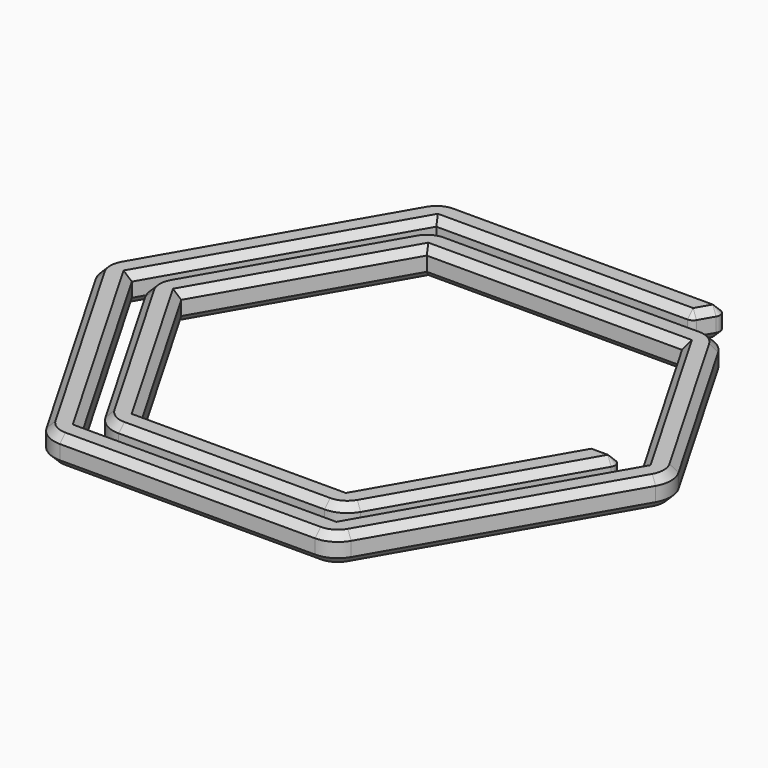
from build123d import *

# Parameters (mm, degrees)
F1_DEPTH = 2
F2_R     = 0.5
F3_R     = 2
F4_SIZE  = 0.49999


# Not quite as in the source:
# - a fillet or chamfer is up to 0.001 mm smaller than in the source, because OpenCascade refuses the exact size


with BuildPart() as f1:
    # F0 (on Top) → F1 (new body)
    with BuildSketch(Plane.XY):
        Polygon((-14.4337567297, 0), (-7.2168783649, 12.5), (7.2168783649, 12.5), (9.5262794416, 12.5), (10.68097998, 12.5), (17.8978583449, 0), (8.9489291724, -15.5), (-8.9489291724, -15.5), (-17.8978583449, 0), (-8.9489291724, 15.5), (8.9489291724, 15.5), (10.1036297108, 17.5), (-10.1036297108, 17.5), (-20.2072594216, 0), (-10.1036297108, -17.5), (10.1036297108, -17.5), (20.2072594216, 0), (11.8356805184, 14.5), (8.3715789032, 14.5), (-8.3715789032, 14.5), (-16.7431578065, 0), (-8.3715789032, -14.5), (8.3715789032, -14.5), (16.7431578065, 0), (14.4337567297, 0), (7.2168783649, -12.5), (-7.2168783649, -12.5), align=None)
    extrude(amount=F1_DEPTH)

    # F2
    f2_edges = [f1.edges().sort_by_distance(p)[0] for p in [
        (16.743158, 0, 1),
        (14.433757, 0, 1),
        (10.10363, 17.5, 1),
        (8.948929, 15.5, 1),
    ]]
    fillet(f2_edges, radius=F2_R)

    # F3
    f3_edges = [f1.edges().sort_by_distance(p)[0] for p in [
        (-10.10363, 17.5, 1),
        (-20.207259, 0, 1),
        (-10.10363, -17.5, 1),
        (10.10363, -17.5, 1),
        (20.207259, 0, 1),
        (11.835681, 14.5, 1),
        (-8.371579, 14.5, 1),
        (-16.743158, 0, 1),
        (-8.371579, -14.5, 1),
        (8.371579, -14.5, 1),
    ]]
    fillet(f3_edges, radius=F3_R)

    # F4 (size 0.5 in the source; OpenCascade refuses exactly that, so slightly less here)
    f4_edges = [f1.edges().sort_by_distance(p)[0] for p in [
        (12.629537, -7.125, 0),
        (8.216878, -14.232051, 0),
        (16.310145, -0.25, 0),
        (0, -14.5, 0),
        (15.299782, 0, 0),
        (-8.216878, -14.232051, 0),
        (14.472432, -0.066987, 0),
        (-12.557368, -7.25, 0),
        (10.753149, -6.375, 0),
        (-16.433757, 0, 0),
        (0, -12.5, 0),
        (-12.557368, 7.25, 0),
        (-10.825318, -6.25, 0),
        (-8.216878, 14.232051, 0),
        (-10.825318, 6.25, 0),
        (1.732051, 14.5, 0),
        (1.732051, 12.5, 0),
        (11.68098, 14.232051, 0),
        (14.289419, 6.25, 0),
        (16.02147, 7.25, 0),
        (13.423394, -7.75, 0),
        (19.897858, 0, 0),
        (0, -15.5, 0),
        (15.155445, -8.75, 0),
        (-13.423394, -7.75, 0),
        (9.948929, -17.232051, 0),
        (-13.423394, 7.75, 0),
        (0, -17.5, 0),
        (-0.144338, 15.5, 0),
        (-9.948929, -17.232051, 0),
        (8.910254, 15.566987, 0),
        (-15.155445, -8.75, 0),
        (9.381942, 16.25, 0),
        (-19.897858, 0, 0),
        (9.670617, 17.25, 0),
        (-15.155445, 8.75, 0),
        (0.144338, 17.5, 0),
        (-9.948929, 17.232051, 0),
        (12.629537, -7.125, 2),
        (8.216878, -14.232051, 2),
        (16.310145, -0.25, 2),
        (0, -14.5, 2),
        (15.299782, 0, 2),
        (-8.216878, -14.232051, 2),
        (14.472432, -0.066987, 2),
        (-12.557368, -7.25, 2),
        (10.753149, -6.375, 2),
        (-16.433757, 0, 2),
        (0, -12.5, 2),
        (-12.557368, 7.25, 2),
        (-10.825318, -6.25, 2),
        (-8.216878, 14.232051, 2),
        (-10.825318, 6.25, 2),
        (1.732051, 14.5, 2),
        (1.732051, 12.5, 2),
        (11.68098, 14.232051, 2),
        (14.289419, 6.25, 2),
        (16.02147, 7.25, 2),
        (13.423394, -7.75, 2),
        (19.897858, 0, 2),
        (0, -15.5, 2),
        (15.155445, -8.75, 2),
        (-13.423394, -7.75, 2),
        (9.948929, -17.232051, 2),
        (-13.423394, 7.75, 2),
        (0, -17.5, 2),
        (-0.144338, 15.5, 2),
        (-9.948929, -17.232051, 2),
        (8.910254, 15.566987, 2),
        (-15.155445, -8.75, 2),
        (9.381942, 16.25, 2),
        (-19.897858, 0, 2),
        (9.670617, 17.25, 2),
        (-15.155445, 8.75, 2),
        (0.144338, 17.5, 2),
        (-9.948929, 17.232051, 2),
    ]]
    chamfer(f4_edges, length=F4_SIZE)


solid = f1.part
